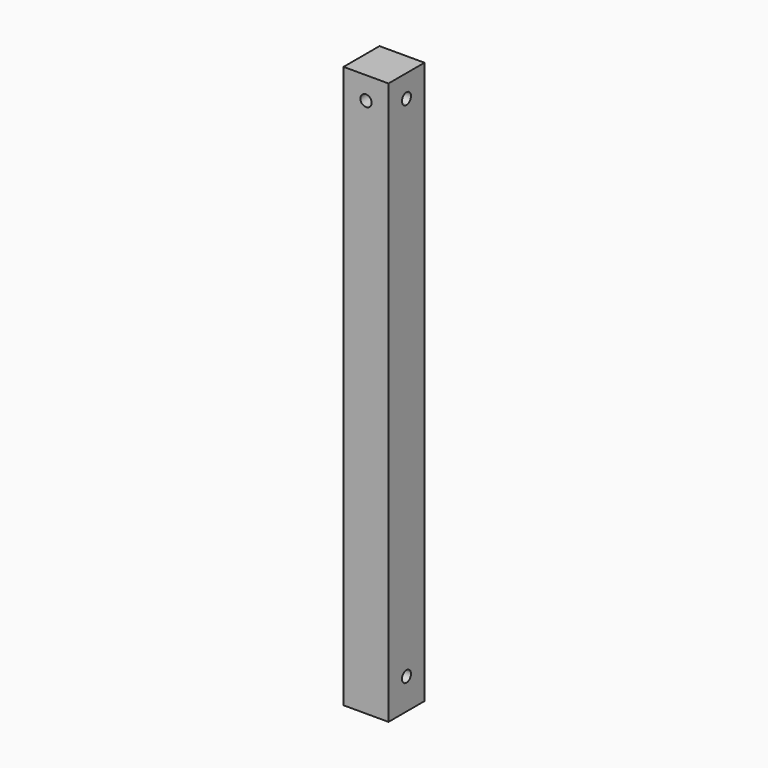
from build123d import *

# Parameters (mm, degrees)
F0_W     = 25.4
F0_H     = 25.4
F1_DEPTH = 304.8
F2_R     = 3.175
F3_DEPTH = 50.8
F4_R     = 3.175
F5_DEPTH = 25.4
F6_R     = 3.175
F7_DEPTH = 25.4
F8_DEPTH = 12.7


with BuildPart() as f1:
    # F0 (on Top) → F1 (new body)
    with BuildSketch(Plane.XY):
        Rectangle(F0_W, F0_H)
    extrude(amount=F1_DEPTH)

    # F2 (on face) → F3 (cut)
    with BuildSketch(Plane.XZ.offset(12.7)):
        with Locations((0, 292.1)):
            Circle(F2_R)
    extrude(amount=-F3_DEPTH, mode=Mode.SUBTRACT)

    # F4 (on face) → F5 (cut)
    with BuildSketch(Plane.YZ.offset(12.7)):
        with Locations((0, 292.1)):
            Circle(F4_R)
    extrude(amount=-F5_DEPTH, mode=Mode.SUBTRACT)

    # F6 (on face) → F7 (cut)
    with BuildSketch(Plane.YZ.offset(12.7)):
        with Locations((0, 4.7888585575)):
            Circle(F6_R)
    extrude(amount=-F7_DEPTH, mode=Mode.SUBTRACT)

    # F8 (add): a face of the model
    f8_faces = [f1.faces().sort_by_distance(p)[0] for p in [
        (0, 0, 0),
    ]]
    extrude(f8_faces, amount=F8_DEPTH)


solid = f1.part
